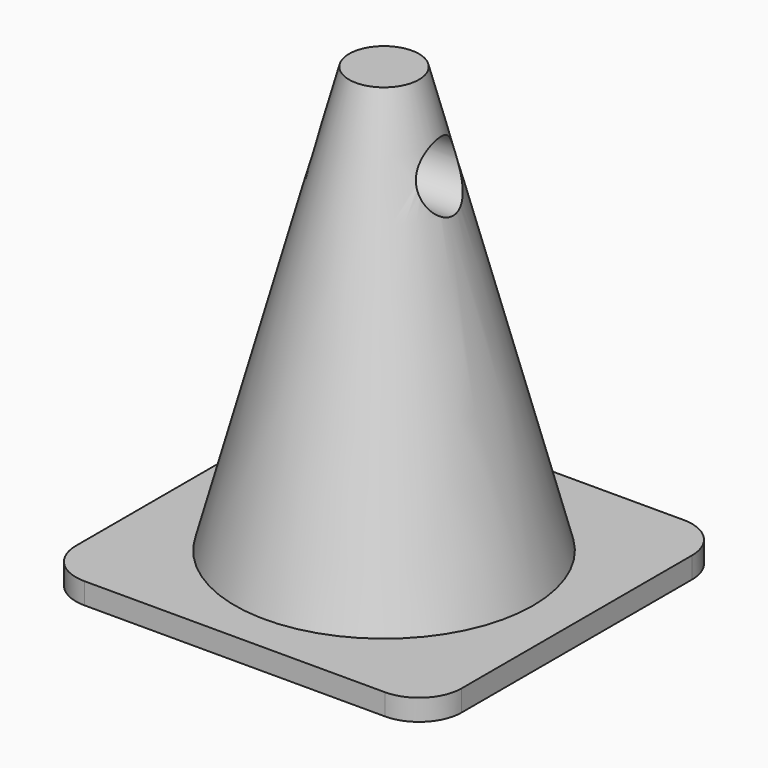
from build123d import *

# Parameters (mm, degrees)
F0_R     = 17.5
F1_DEPTH = 2.5
F2_R     = 17.5
F3_DEPTH = 50
F3_TAPER = 15
F4_R     = 3.6137849114
F5_DEPTH = 60
F6_R     = 13.2346261553


# Not quite as in the source:
# - an extrude whose draft closes it to a point is written as a loft to that point


with BuildPart() as f1:
    # F0 (on Top) → F1 (new body)
    with BuildSketch(Plane.XY):
        with BuildLine():
            Line((0, 38.8068709316), (-35.2930977718, 38.8068709316))
            ThreePointArc((-35.2930977718, 38.8068709316), (-38.8286316778, 37.3424048375), (-40.2930977718, 33.8068709316))
            Line((-40.2930977718, 33.8068709316), (-40.2930977718, 0))
            ThreePointArc((-40.2930977718, 0), (-38.8286316778, -3.5355339059), (-35.2930977718, -5))
            Line((-35.2930977718, -5), (0, -5))
            ThreePointArc((0, -5), (3.5355339059, -3.5355339059), (5, 0))
            Line((5, 0), (5, 33.8068709316))
            ThreePointArc((5, 33.8068709316), (3.5355339059, 37.3424048375), (0, 38.8068709316))
        make_face()
        with Locations((-17.6465488859, 16.9034354658)):
            Circle(F0_R, mode=Mode.SUBTRACT)
        with Locations((-17.6465488859, 16.9034354658)):
            Circle(F0_R)
    extrude(amount=F1_DEPTH)

    # F2 (on face) → F3 (join)
    with BuildSketch(Plane.XY.offset(2.5)):
        with Locations((-17.6465488859, 16.9034354658)):
            Circle(F2_R)
    extrude(amount=F3_DEPTH, taper=F3_TAPER)

    # F4 (on Right) → F5 (cut)
    with BuildSketch(Plane.YZ):
        with Locations((17.7631601691, 42.927633971)):
            Circle(F4_R)
    extrude(amount=-F5_DEPTH, mode=Mode.SUBTRACT)

    # F6 (on face) → F7 section 0
    with BuildSketch(Plane(origin=(0, 0, 0), x_dir=(1, 0, 0), z_dir=(0, 0, -1)), mode=Mode.PRIVATE) as f7_s0:
        with Locations((-17.6465488859, -16.9034354658)):
            Circle(F6_R)
    loft([f7_s0.sketch, Vertex(-17.6465488859, 16.9034354658, 22.9230449201)], ruled=True, mode=Mode.SUBTRACT)


solid = f1.part
